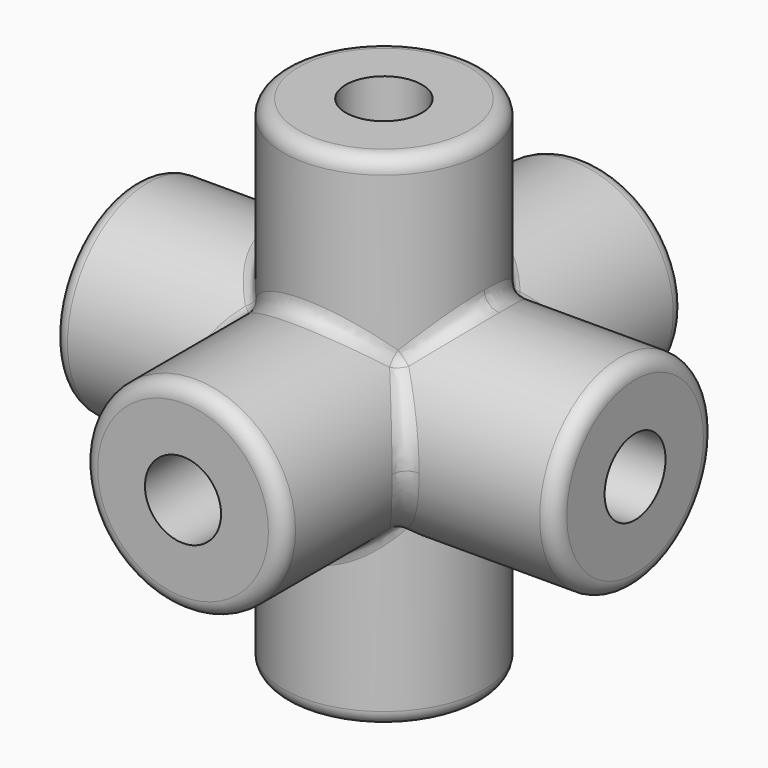
from build123d import *

# Parameters (mm, degrees)
F0_R     = 5.08
F0_R_2   = 1.925
F1_DEPTH = 12.7
F2_R     = 5.08
F2_R_2   = 1.925
F4_DEPTH = 12.7
F3_R     = 5.08
F3_R_2   = 1.925
F5_DEPTH = 12.7
F6_R     = 0.762


with BuildPart() as f1:
    # F0 (on Front) → F1 (new body, symmetric)
    with BuildSketch(Plane.XZ):
        Circle(F0_R)
        Circle(F0_R_2, mode=Mode.SUBTRACT)
    extrude(amount=F1_DEPTH, both=True)

    # F2 (on Right) → F4 (join, symmetric)
    with BuildSketch(Plane.YZ):
        Circle(F2_R)
        Circle(F2_R_2, mode=Mode.SUBTRACT)
    extrude(amount=F4_DEPTH, both=True)

    # F3 (on Top) → F5 (join, symmetric)
    with BuildSketch(Plane.XY):
        Circle(F3_R)
        Circle(F3_R_2, mode=Mode.SUBTRACT)
    extrude(amount=F5_DEPTH, both=True)

    # F6
    f6_edges = [f1.edges().sort_by_distance(p)[0] for p in [
        (-5.08, 0, 12.7),
        (-5.08, -12.7, 0),
        (12.7, -5.08, 0),
        (-5.08, 12.7, 0),
        (-5.08, 0, -12.7),
        (-12.7, -5.08, 0),
        (0, 5.08, 5.08),
        (0, 5.08, -5.08),
        (-5.08, 0, 5.08),
        (-5.08, 0, -5.08),
        (4.649244, 4.649244, 2.047175),
        (-4.649244, 4.649244, 2.047175),
        (-4.649244, 4.649244, -2.047175),
        (4.649244, 4.649244, -2.047175),
        (-4.649244, -4.649244, -2.047175),
        (-4.649244, -4.649244, 2.047175),
        (4.649244, -4.649244, 2.047175),
        (4.649244, -4.649244, -2.047175),
        (-2.047175, -4.649244, 4.649244),
        (2.047175, -4.649244, 4.649244),
        (2.047175, -4.649244, -4.649244),
        (-2.047175, -4.649244, -4.649244),
        (4.693308, -1.944032, 4.693308),
        (4.693308, 1.944032, 4.693308),
    ]]
    fillet(f6_edges, radius=F6_R)


solid = f1.part
